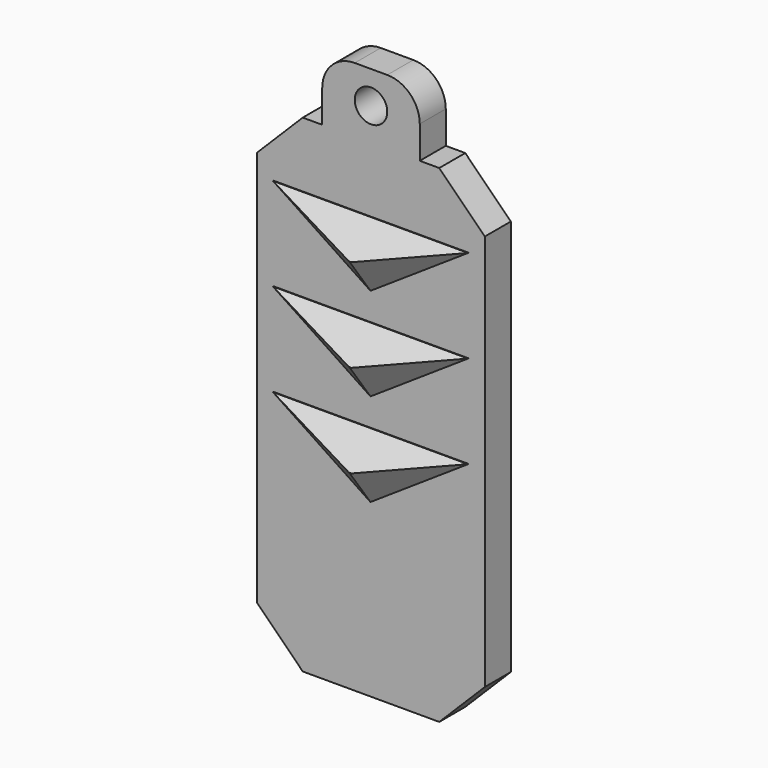
from build123d import *

# Parameters (mm, degrees)
F0_R       = 2.5
F1_DEPTH   = 5
F2_SIZE    = 7
F3_DEPTH   = 10
F4_R       = 5
F5_DEPTH   = 9
F6_SIZE2   = 3.9
F6_SIZE    = 4.4864367882
F6_2_SIZE2 = 3.9
F6_2_SIZE  = 4.4864367882
F6_3_SIZE2 = 3.9
F6_3_SIZE  = 4.4864367882


# Not quite as in the source:
# - a feature names something its author has since deleted; it is built from what else it names


with BuildPart() as f1:
    # F0 (on Front) → F1 (new body)
    with BuildSketch(Plane.XZ):
        Polygon((17.5, -37.5), (17.5, 37.5), (7.5, 37.5), (0, 37.5), (-7.5, 37.5), (-17.5, 37.5), (-17.5, -37.5), align=None)
        Polygon((0, -11.1), (-15, -1.1), (15, -1.1), align=None, mode=Mode.SUBTRACT)
        Polygon((0, 3.2), (-15, 13.2), (15, 13.2), align=None, mode=Mode.SUBTRACT)
        Polygon((0, 17.5), (-15, 27.5), (15, 27.5), align=None, mode=Mode.SUBTRACT)
        Polygon((0, 37.5), (7.5, 37.5), (7.5, 47.5), (0, 47.5), (-7.5, 47.5), (-7.5, 37.5), align=None)
        with Locations((0, 42.5)):
            Circle(F0_R, mode=Mode.SUBTRACT)
    extrude(amount=F1_DEPTH)

    # F2
    f2_edges = [f1.edges().sort_by_distance(p)[0] for p in [
        (-17.5, -2.5, 37.5),
        (17.5, -2.5, 37.5),
        (-17.5, -2.5, -37.5),
        (17.5, -2.5, -37.5),
    ]]
    chamfer(f2_edges, length=F2_SIZE)

    # F0 (on Front) → F3 (cut)
    with BuildSketch(Plane.XZ):
        with Locations((0, 42.5)):
            Circle(F0_R)
    extrude(amount=-F3_DEPTH, mode=Mode.SUBTRACT)

    # F4
    f4_edges = [f1.edges().sort_by_distance(p)[0] for p in [
        (-7.5, -2.5, 47.5),
        (7.5, -2.5, 47.5),
    ]]
    fillet(f4_edges, radius=F4_R)

    # F0 (on Front) → F5 (join)
    with BuildSketch(Plane.XZ):
        Polygon((15, 27.5), (-15, 27.5), (0, 17.5), align=None)
        Polygon((15, 13.2), (-15, 13.2), (0, 3.2), align=None)
        Polygon((15, -1.1), (-15, -1.1), (0, -11.1), align=None)
    extrude(amount=F5_DEPTH)

    # F6
    f6_edges = [f1.edges().sort_by_distance(p)[0] for p in [
        (0, -9, -1.1),
        (-7.5, -9, -6.1),
        (7.5, -9, -6.1),
    ]]
    f6_side = f1.faces().sort_by_distance((0, -9, -4.433333))[0]
    chamfer(f6_edges, length=F6_SIZE, length2=F6_SIZE2, reference=f6_side)

    # F6#2
    f6_2_edges = [f1.edges().sort_by_distance(p)[0] for p in [
        (0, -9, 13.2),
        (-7.5, -9, 8.2),
        (7.5, -9, 8.2),
    ]]
    f6_2_side = f1.faces().sort_by_distance((0, -9, 9.866667))[0]
    chamfer(f6_2_edges, length=F6_2_SIZE, length2=F6_2_SIZE2, reference=f6_2_side)

    # F6#3
    f6_3_edges = [f1.edges().sort_by_distance(p)[0] for p in [
        (0, -9, 27.5),
        (-7.5, -9, 22.5),
        (7.5, -9, 22.5),
    ]]
    f6_3_side = f1.faces().sort_by_distance((0, -9, 24.166667))[0]
    chamfer(f6_3_edges, length=F6_3_SIZE, length2=F6_3_SIZE2, reference=f6_3_side)


solid = f1.part
